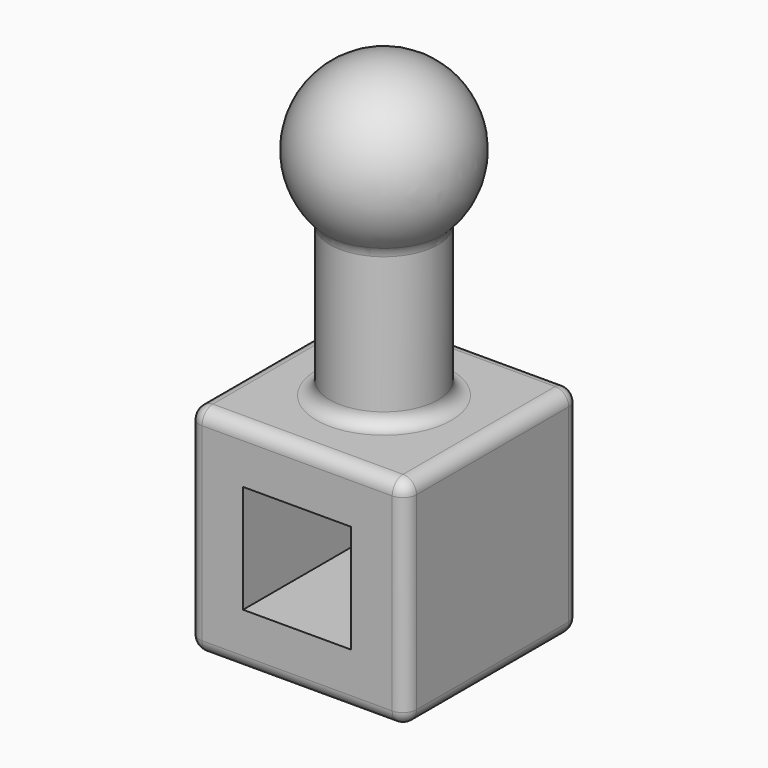
from build123d import *

# Parameters (mm, degrees)
F0_W     = 102.0282506943
F0_H     = 102.0282581449
F1_DEPTH = 101.6
F2_R     = 25.4
F3_DEPTH = 101.6
F6_W     = 50.8
F6_H     = 50.8
F7_DEPTH = 130.048
F8_R     = 6.35


with BuildPart() as f1:
    # F0 (on Top) → F1 (new body)
    with BuildSketch(Plane.XY):
        Rectangle(F0_W, F0_H)
    extrude(amount=F1_DEPTH)

    # F2 (on face) → F3 (join)
    with BuildSketch(Plane.XY.offset(101.6)):
        Circle(F2_R)
    extrude(amount=F3_DEPTH)

    # F4 (on face) → F5 (revolve)
    with BuildSketch(Plane.XY.offset(203.2)):
        with BuildLine():
            Line((0, -25.4), (0, -38.1))
            ThreePointArc((0, -38.1), (38.1, 0), (0, 38.1))
            Line((0, 38.1), (0, 25.4))
            ThreePointArc((0, 25.4), (17.9605122421, 17.9605122421), (25.4, 0))
            ThreePointArc((25.4, 0), (17.9605122421, -17.9605122421), (0, -25.4))
        make_face()
        with BuildLine():
            ThreePointArc((0, 25.4), (-25.4, 0), (0, -25.4))
            Line((0, -25.4), (0, 0))
            Line((0, 0), (0, 25.4))
        make_face()
    revolve(axis=Axis((0, 0, 203.2), (0, -1, 0)))

    # F6 (on face) → F7 (cut)
    with BuildSketch(Plane.XZ.offset(51.0141290724)):
        with Locations((0, 50.8)):
            Rectangle(F6_W, F6_H)
    extrude(amount=-F7_DEPTH, mode=Mode.SUBTRACT)

    # F8
    f8_edges = [f1.edges().sort_by_distance(p)[0] for p in [
        (51.014125, 0, 101.6),
        (51.014125, -51.014129, 50.8),
        (51.014125, 0, 0),
        (51.014125, 51.014129, 50.8),
        (0, -51.014129, 101.6),
        (0, -51.014129, 0),
        (-51.014125, -51.014129, 50.8),
        (-51.014125, 0, 101.6),
        (0, 51.014129, 101.6),
        (-51.014125, 51.014129, 50.8),
        (0, 51.014129, 0),
        (-51.014125, 0, 0),
        (-25.4, 0, 101.6),
        (-25.4, 0, 174.801937),
    ]]
    fillet(f8_edges, radius=F8_R)


solid = f1.part
